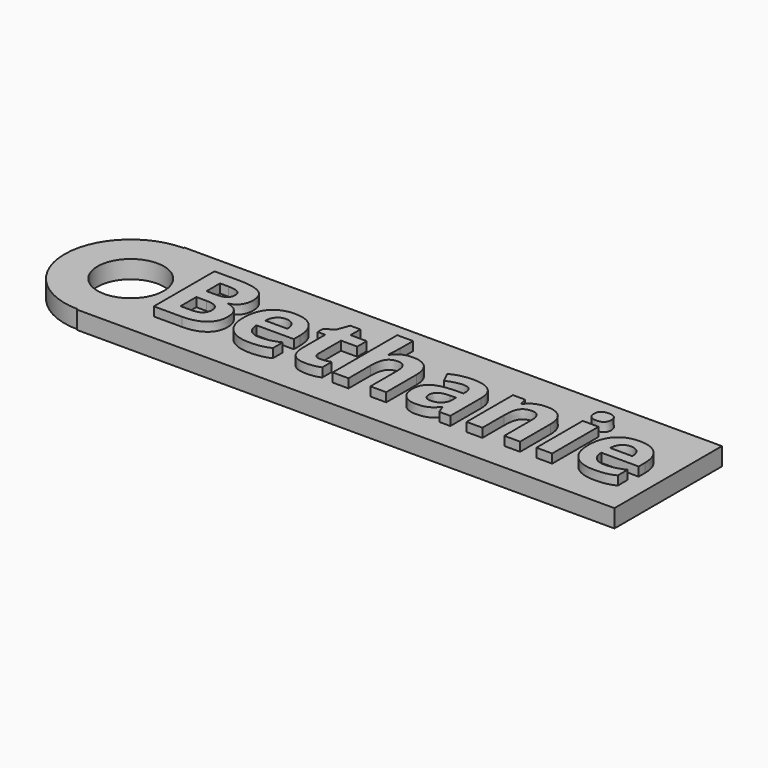
from build123d import *

# Parameters (mm, degrees)
F0_R         = 3.7051787774
F1_DEPTH     = 2
F2_TEXT_SIZE = 11.8519114848
F3_DEPTH     = 1


# Not quite as in the source:
# - Text() gives the source's letters only with a copy of the font that has no kerning and outlines rounded to 1/6400 em; it was checked with that copy


with BuildPart() as f1:
    # F0 (on Top) → F1 (new body)
    with BuildSketch(Plane.XY):
        with BuildLine():
            Line((44.2340736836, -4.8621181054), (-15.7659263164, -4.8621181054))
            Line((-15.7659263164, -4.8621181054), (-15.7659263164, -4.9716483758))
            ThreePointArc((-15.7659263164, -4.9716483758), (-23.156396046, -12.3621181054), (-15.7659263164, -19.7525878349))
            Line((-15.7659263164, -19.7525878349), (-15.7659263164, -19.8621181054))
            Line((-15.7659263164, -19.8621181054), (44.2340736836, -19.8621181054))
            Line((44.2340736836, -19.8621181054), (44.2340736836, -4.8621181054))
        make_face()
        with Locations((-15.7659263164, -12.3621181054)):
            Circle(F0_R, mode=Mode.SUBTRACT)
    extrude(amount=F1_DEPTH)

    # F2 (on face) → F3 (join)
    with BuildSketch(Plane.XY.offset(2)):
        with Locations((-10.7878129929, -16.6945476085)):
            Text('Bethanie', F2_TEXT_SIZE, font='Open Sans', font_style=FontStyle.BOLD, text_align=(TextAlign.LEFT, TextAlign.BOTTOM))
    extrude(amount=F3_DEPTH)


solid = f1.part
